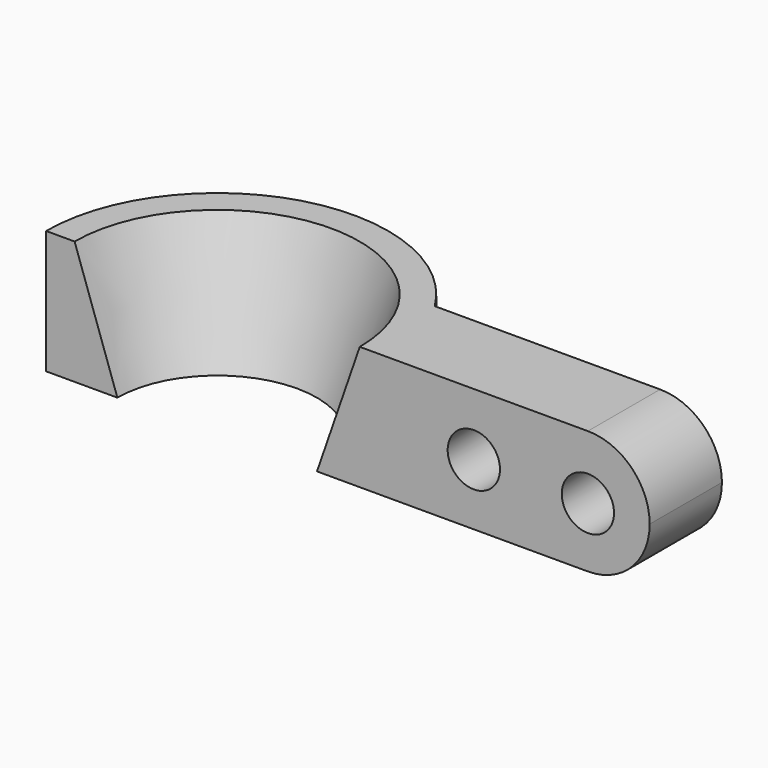
from build123d import *

# Parameters (mm, degrees)
F1_DEPTH = 52
F4_R     = 11
F5_DEPTH = 38
F6_R     = 25.99999


# Not quite as in the source:
# - a fillet or chamfer is up to 0.001 mm smaller than in the source, because OpenCascade refuses the exact size


with BuildPart() as f1:
    # F0 (on Top) → F1 (new body)
    with BuildSketch(Plane.XY):
        with BuildLine():
            Line((182, 38), (61.1555394057, 38))
            ThreePointArc((61.1555394057, 38), (-19.7585571689, 69.2358246763), (-72, 0))
            Line((-72, 0), (182, 0))
            Line((182, 0), (182, 38))
        make_face()
    extrude(amount=F1_DEPTH)

    # F2 (on face) → F3 (revolve, cut)
    with BuildSketch(Plane.XZ):
        Polygon((60, 52), (0, 52), (0, 0), (42, 0), align=None)
    revolve(axis=Axis((0, 0, 26), (0, 0, -1)), mode=Mode.SUBTRACT)

    # F4 (on face) → F5 (cut)
    with BuildSketch(Plane.XZ):
        with Locations((108, 25.7937852293)):
            Circle(F4_R)
        with Locations((156, 25.2048280338)):
            Circle(F4_R)
    extrude(amount=-F5_DEPTH, mode=Mode.SUBTRACT)

    # F6 (radius 26 in the source; OpenCascade refuses exactly that, so slightly less here)
    f6_edges = [f1.edges().sort_by_distance(p)[0] for p in [
        (182, 19, 52),
        (182, 19, 0),
    ]]
    fillet(f6_edges, radius=F6_R)


solid = f1.part
